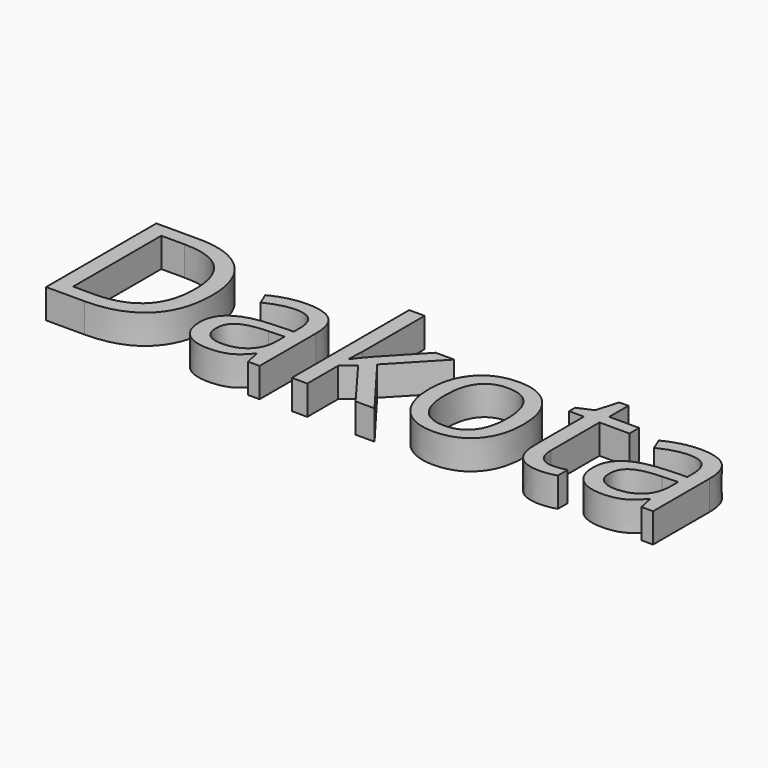
from build123d import *

# Parameters (mm, degrees)
F0_TEXT_SIZE = 167.0076770501
F1_DEPTH     = 25.4


# Not quite as in the source:
# - Text() gives the source's letters only with a copy of the font that has no kerning and outlines rounded to 1/6400 em; it was checked with that copy


with BuildPart() as f1:
    # F0 (on Top) → F1 (new body)
    with BuildSketch(Plane.XY):
        with Locations((-234.3308255076, -109.129470773)):
            Text('Dakota', F0_TEXT_SIZE, font='Open Sans', text_align=(TextAlign.LEFT, TextAlign.BOTTOM))
    extrude(amount=F1_DEPTH)


solid = f1.part
